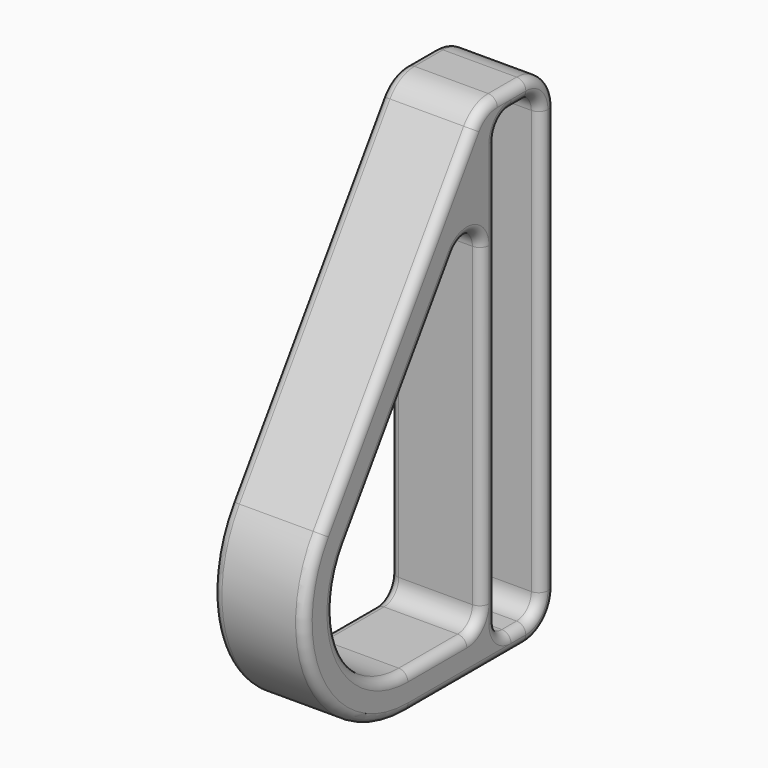
from build123d import *

# Parameters (mm, degrees)
F2_W     = 10
F2_H     = 54
F2_W_2   = 6
F2_H_2   = 50
F3_DEPTH = 5
F5_DEPTH = 5
F6_R     = 4
F7_R     = 2
F8_R     = 0.99999


# Not quite as in the source:
# - a fillet or chamfer is up to 0.001 mm smaller than in the source, because OpenCascade refuses the exact size


with BuildPart() as f3:
    # F2 (on Right) → F3 (new body, symmetric)
    with BuildSketch(Plane.YZ):
        with Locations((5, 27)):
            Rectangle(F2_W, F2_H)
        with Locations((5, 27)):
            Rectangle(F2_W_2, F2_H_2, mode=Mode.SUBTRACT)
    extrude(amount=F3_DEPTH, both=True)

    # F4 (on Right) → F5 (join, symmetric)
    with BuildSketch(Plane.YZ):
        with BuildLine():
            Line((0, 0), (0, 4))
            Line((0, 4), (-10, 4))
            ThreePointArc((-10, 4), (-18.824788597, 9.2964793805), (-18.3015150257, 19.5753787564))
            Line((-18.3015150257, 19.5753787564), (0, 46.8255995247))
            Line((0, 46.8255995247), (0, 54))
            Line((0, 54), (-21.622121036, 21.805530259))
            ThreePointArc((-21.622121036, 21.805530259), (-22.3547040358, 7.4150711327), (-10, 0))
            Line((-10, 0), (0, 0))
        make_face()
    extrude(amount=F5_DEPTH, both=True)

    # F6
    f6_edges = [f3.edges().sort_by_distance(p)[0] for p in [
        (0, 10, 54),
        (0, 0, 54),
        (0, 10, 0),
    ]]
    fillet(f6_edges, radius=F6_R)

    # F7
    f7_edges = [f3.edges().sort_by_distance(p)[0] for p in [
        (0, 8, 52),
        (0, 2, 52),
        (0, 8, 2),
        (0, 2, 2),
        (0, 0, 4),
        (0, 0, 46.8256),
    ]]
    fillet(f7_edges, radius=F7_R)

    # F8 (radius 1 in the source; OpenCascade refuses exactly that, so slightly less here)
    f8_edges = [f3.edges().sort_by_distance(p)[0] for p in [
        (5, 0, 23.13024),
        (5, -1.417165, 42.173671),
        (5, -0.585786, 4.585786),
        (5, -10.980909, 30.475467),
        (5, -6, 4),
        (5, -18.824789, 9.296479),
        (5, 4.065979, 54),
        (5, 8.828427, 52.828427),
        (5, 0.25055, 53.529915),
        (5, 10, 27),
        (5, -11.405384, 37.017841),
        (5, 8.828427, 1.171573),
        (5, -22.354704, 7.415071),
        (5, -2, 0),
        (5, 8, 27),
        (5, 7.414214, 51.414214),
        (5, 7.414214, 2.585786),
        (5, 5, 52),
        (5, 5, 2),
        (5, 2.585786, 51.414214),
        (5, 2.585786, 2.585786),
        (5, 2, 27),
        (-5, 0, 23.13024),
        (-5, -1.417165, 42.173671),
        (-5, -0.585786, 4.585786),
        (-5, -10.980909, 30.475467),
        (-5, -6, 4),
        (-5, -18.824789, 9.296479),
        (-5, 4.065979, 54),
        (-5, 8.828427, 52.828427),
        (-5, 0.25055, 53.529915),
        (-5, 10, 27),
        (-5, -11.405384, 37.017841),
        (-5, 8.828427, 1.171573),
        (-5, -22.354704, 7.415071),
        (-5, -2, 0),
        (-5, 8, 27),
        (-5, 7.414214, 51.414214),
        (-5, 7.414214, 2.585786),
        (-5, 5, 52),
        (-5, 5, 2),
        (-5, 2.585786, 51.414214),
        (-5, 2.585786, 2.585786),
        (-5, 2, 27),
    ]]
    fillet(f8_edges, radius=F8_R)


solid = f3.part
